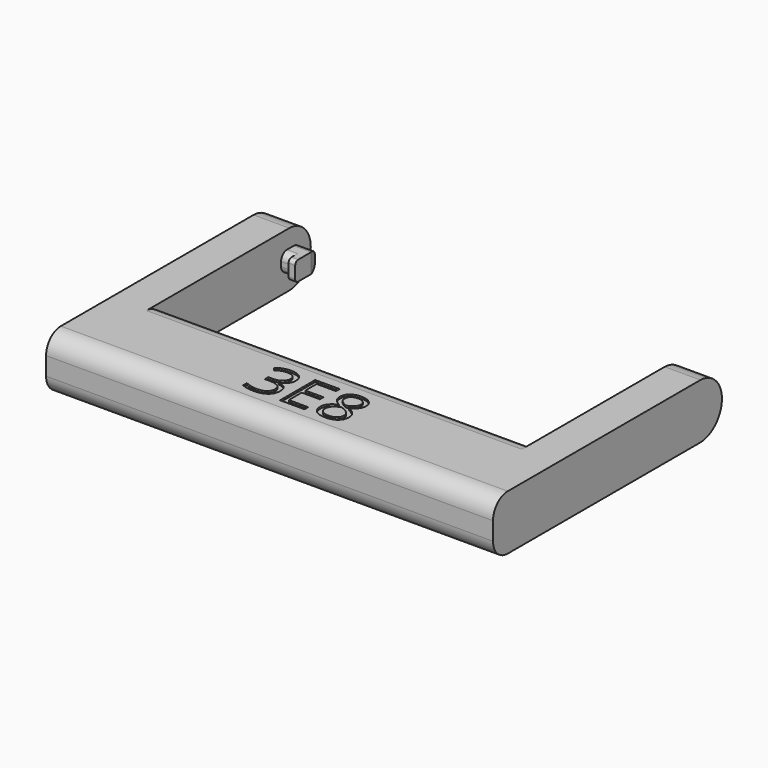
from build123d import *

# Parameters (mm, degrees)
F0_W          = 121.2
F0_H          = 77.6
F1_DEPTH      = 14.9
F2_W          = 101.8
F2_H          = 50.7
F3_DEPTH      = 14.901
F5_DEPTH      = 9.701
F5_DEPTH_BACK = 111.501
F6_R          = 5
F7_W          = 7.4
F7_H          = 5.25
F8_DEPTH      = 101.8
F9_W          = 92.4
F9_H          = 7.4
F9_W_2        = 2.9
F9_H_2        = 1.1
F10_DEPTH     = 10.076
F11_R         = 2
F12_R         = 1
F14_DEPTH     = 10.076
F15_TEXT_SIZE = 16.6666666667
F16_DEPTH     = 0.5


# Not quite as in the source:
# - Text() gives the source's letters only with a copy of the font that has no kerning and outlines rounded to 1/6400 em; it was checked with that copy


with BuildPart() as f1:
    # F0 (on Top) → F1 (new body)
    with BuildSketch(Plane.XY):
        Rectangle(F0_W, F0_H)
    extrude(amount=F1_DEPTH)

    # F2 (on face) → F3 (cut, through all)
    with BuildSketch(Plane.XY.offset(14.9)):
        with Locations((0, 13.45)):
            Rectangle(F2_W, F2_H)
    extrude(amount=-F3_DEPTH, mode=Mode.SUBTRACT)

    # F4 (on face) → F5 (cut, two sides)
    with BuildSketch(Plane.YZ.offset(-50.9)) as f5_sk:
        with BuildLine():
            Line((31.512071555, 0), (38.8, 0))
            Line((38.8, 0), (38.8, 7.45))
            ThreePointArc((38.8, 7.45), (36.6750407073, 2.239040371), (31.512071555, 0))
        make_face()
        with BuildLine():
            ThreePointArc((31.1843242399, 0), (31.3481978974, -0.0018021026), (31.512071555, 0))
            Line((31.512071555, 0), (31.1843242399, 0))
        make_face()
        with BuildLine():
            ThreePointArc((31.512071555, 14.9), (36.6750407073, 12.660959629), (38.8, 7.45))
            Line((38.8, 7.45), (38.8, 14.9))
            Line((38.8, 14.9), (31.512071555, 14.9))
        make_face()
    extrude(amount=-F5_DEPTH, mode=Mode.SUBTRACT)
    extrude(f5_sk.sketch, amount=F5_DEPTH_BACK, mode=Mode.SUBTRACT)

    # F6
    f6_edges = [f1.edges().sort_by_distance(p)[0] for p in [
        (0, -11.9, 14.9),
        (0, -11.9, 0),
        (0, -38.8, 14.9),
        (0, -38.8, 0),
    ]]
    fillet(f6_edges, radius=F6_R)

    # F7 (on face) → F8 (join, through all)
    with BuildSketch(Plane.YZ.offset(-50.9)):
        with Locations((31.3481978974, 7.45)):
            Rectangle(F7_W, F7_H)
    extrude(amount=F8_DEPTH)

    # F9 (on face) → F10 (cut, through all)
    with BuildSketch(Plane.XY.offset(10.075)):
        with Locations((0, 31.3481978974)):
            Rectangle(F9_W, F9_H)
        with Locations((-49.45, 28.1981978974)):
            Rectangle(F9_W_2, F9_H_2)
        with Locations((49.45, 28.1981978974)):
            Rectangle(F9_W_2, F9_H_2)
    extrude(amount=-F10_DEPTH, mode=Mode.SUBTRACT)

    # F11
    f11_edges = [f1.edges().sort_by_distance(p)[0] for p in [
        (-48.55, 35.048198, 10.075),
        (-48.55, 35.048198, 4.825),
        (-49.45, 28.748198, 10.075),
        (-49.45, 28.748198, 4.825),
        (49.45, 28.748198, 10.075),
        (48.55, 35.048198, 10.075),
        (48.55, 35.048198, 4.825),
        (49.45, 28.748198, 4.825),
    ]]
    fillet(f11_edges, radius=F11_R)

    # F12
    f12_edges = [f1.edges().sort_by_distance(p)[0] for p in [
        (-47.1, 27.648198, 4.825),
        (-47.1, 27.648198, 10.075),
        (47.1, 27.648198, 4.825),
        (47.1, 27.648198, 10.075),
    ]]
    fillet(f12_edges, radius=F12_R)

    # F13 (on face) → F14 (cut, through all)
    with BuildSketch(Plane(origin=(0, 0, 4.825), x_dir=(1, 0, 0), z_dir=(0, 0, -1))):
        Polygon((-46.7358983849, -35.0481978974), (-46.2, -35.0481978974), (-46.2, -33.0481978974), align=None)
        Polygon((46.2, -33.0481978974), (46.2, -35.0481978974), (46.7358983849, -35.0481978974), align=None)
    extrude(amount=-F14_DEPTH, mode=Mode.SUBTRACT)

    # F15 (on face) → F16 (cut)
    with BuildSketch(Plane.XY.offset(14.9)):
        with Locations((-14.2721354167, -31.35)):
            Text('3E8', F15_TEXT_SIZE, font='Open Sans', text_align=(TextAlign.LEFT, TextAlign.BOTTOM))
    extrude(amount=-F16_DEPTH, mode=Mode.SUBTRACT)


solid = f1.part
